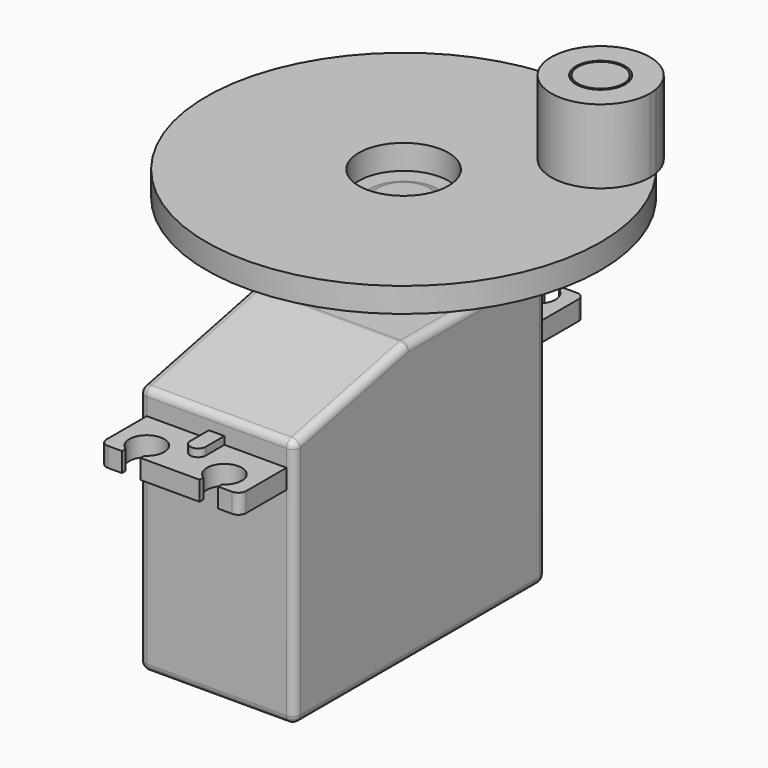
from build123d import *

# Parameters (mm, degrees)
F1_DEPTH  = 10
F0_W      = 7.5
F0_H      = 2.5
F2_DEPTH  = 9
F4_DEPTH  = 25
F5_W      = 2
F5_H      = 46.5
F6_DEPTH  = 1
F9_R      = 0.8128
F10_DEPTH = 2
F11_R     = 26.294756744
F12_DEPTH = 2
F13_R     = 0.99999
F14_R     = 25.4
F14_R_2   = 5.77
F15_DEPTH = 3.175
F16_R     = 2.921
F17_DEPTH = 9.525
F18_R     = 3.175
F19_DEPTH = 9.525


# Not quite as in the source:
# - a fillet or chamfer is up to 0.001 mm smaller than in the source, because OpenCascade refuses the exact size


with BuildPart() as f1:
    # F0 (on Right) → F1 (new body, symmetric)
    with BuildSketch(Plane.YZ):
        Polygon((-20.25, 26.6), (-20.25, 0), (20.25, 0), (20.25, 26.6), (20.25, 29.1), (20.25, 36.1), (-1.95, 36.1), (-20.25, 32.1), (-20.25, 29.1), align=None)
    extrude(amount=F1_DEPTH, both=True)

    # F0 (on Right) → F2 (join, symmetric)
    with BuildSketch(Plane.YZ):
        with Locations((-24, 27.85)):
            Rectangle(F0_W, F0_H)
        with Locations((24, 27.85)):
            Rectangle(F0_W, F0_H)
    extrude(amount=F2_DEPTH, both=True)

    # F3 (on face) → F4 (cut)
    with BuildSketch(Plane.XY.offset(29.1)):
        with BuildLine():
            ThreePointArc((-3.8, -27.1532866311), (-3.0299111695, -26.336853256), (-2.75, -25.25))
            ThreePointArc((-2.75, -25.25), (-6.086853256, -23.2799111695), (-6.2, -27.1532866311))
            ThreePointArc((-6.2, -27.1532866311), (-5, -27.5), (-3.8, -27.1532866311))
        make_face()
        with BuildLine():
            ThreePointArc((-3.8, -27.1532866311), (-5, -27.5), (-6.2, -27.1532866311))
            Line((-6.2, -27.1532866311), (-6.2, -27.75))
            Line((-6.2, -27.75), (-3.8, -27.75))
            Line((-3.8, -27.75), (-3.8, -27.1532866311))
        make_face()
        with BuildLine():
            Line((-3.8, 27.75), (-6.2, 27.75))
            Line((-6.2, 27.75), (-6.2, 27.1532866311))
            ThreePointArc((-6.2, 27.1532866311), (-5, 27.5), (-3.8, 27.1532866311))
            Line((-3.8, 27.1532866311), (-3.8, 27.75))
        make_face()
        with BuildLine():
            ThreePointArc((-3.8, 27.1532866311), (-5, 27.5), (-6.2, 27.1532866311))
            ThreePointArc((-6.2, 27.1532866311), (-6.086853256, 23.2799111695), (-2.75, 25.25))
            ThreePointArc((-2.75, 25.25), (-3.0299111695, 26.336853256), (-3.8, 27.1532866311))
        make_face()
        with BuildLine():
            Line((3.8, -27.1532866311), (3.8, -27.75))
            Line((3.8, -27.75), (6.2, -27.75))
            Line((6.2, -27.75), (6.2, -27.1532866311))
            ThreePointArc((6.2, -27.1532866311), (5, -27.5), (3.8, -27.1532866311))
        make_face()
        with BuildLine():
            ThreePointArc((7.25, -25.25), (3.913146744, -23.2799111695), (3.8, -27.1532866311))
            ThreePointArc((3.8, -27.1532866311), (5, -27.5), (6.2, -27.1532866311))
            ThreePointArc((6.2, -27.1532866311), (6.9700888305, -26.336853256), (7.25, -25.25))
        make_face()
        with BuildLine():
            Line((6.2, 27.75), (3.8, 27.75))
            Line((3.8, 27.75), (3.8, 27.1532866311))
            ThreePointArc((3.8, 27.1532866311), (5, 27.5), (6.2, 27.1532866311))
            Line((6.2, 27.1532866311), (6.2, 27.75))
        make_face()
        with BuildLine():
            ThreePointArc((6.2, 27.1532866311), (5, 27.5), (3.8, 27.1532866311))
            ThreePointArc((3.8, 27.1532866311), (3.913146744, 23.2799111695), (7.25, 25.25))
            ThreePointArc((7.25, 25.25), (6.9700888305, 26.336853256), (6.2, 27.1532866311))
        make_face()
    extrude(amount=-F4_DEPTH, mode=Mode.SUBTRACT)

    # F5 (on face) → F6 (join)
    with BuildSketch(Plane.XY.offset(29.1)):
        Rectangle(F5_W, F5_H)
        with BuildLine():
            Line((-1, 23.25), (1, 23.25))
            ThreePointArc((1, 23.25), (0, 24.25), (-1, 23.25))
        make_face()
        with BuildLine():
            ThreePointArc((-1, -23.25), (0, -24.25), (1, -23.25))
            Line((1, -23.25), (-1, -23.25))
        make_face()
    extrude(amount=F6_DEPTH)

    # F7 (on Right) → F8 (revolve)
    with BuildSketch(Plane.YZ):
        Polygon((9.85, 36.1), (16.85, 36.1), (13.85, 37.6), (13.85, 42.1), (29.85, 42.1), (29.85, 44.1), (14.35, 44.1), (13.1, 44.6), (9.85, 44.6), align=None)
    revolve(axis=Axis((0, 9.85, 38.956922479), (0, 0, -1)))

    # F9 (on face) → F10 (cut, through all)
    with BuildSketch(Plane.XY.offset(44.1)):
        with Locations((0, 17.3)):
            Circle(F9_R)
        with Locations((0, 20.3)):
            Circle(F9_R)
        with Locations((0, 23.3)):
            Circle(F9_R)
        with Locations((0, 26.3)):
            Circle(F9_R)
        with Locations((-16.45, 9.85)):
            Circle(F9_R)
        with Locations((-13.45, 9.85)):
            Circle(F9_R)
        with Locations((-10.45, 9.85)):
            Circle(F9_R)
        with Locations((-7.45, 9.85)):
            Circle(F9_R)
        with Locations((0, -6.6)):
            Circle(F9_R)
        with Locations((0, -3.6)):
            Circle(F9_R)
        with Locations((0, -0.6)):
            Circle(F9_R)
        with Locations((0, 2.4)):
            Circle(F9_R)
        with Locations((16.45, 9.85)):
            Circle(F9_R)
        with Locations((13.45, 9.85)):
            Circle(F9_R)
        with Locations((10.45, 9.85)):
            Circle(F9_R)
        with Locations((7.45, 9.85)):
            Circle(F9_R)
    extrude(amount=-F10_DEPTH, mode=Mode.SUBTRACT)

    # F11 (on face) → F12 (cut, through all)
    with BuildSketch(Plane.XY.offset(44.1)):
        with Locations((0, 9.85)):
            Circle(F11_R)
        with BuildLine():
            ThreePointArc((-4.8436814511, 14.6936814511), (-4.0616110554, 15.7958081166), (-3.6873277698, 17.0943570425))
            Line((-3.6873277698, 17.0943570425), (-2.5, 27.6162423281))
            ThreePointArc((-2.5, 27.6162423281), (-1.6762811024, 29.2102108544), (0, 29.85))
            ThreePointArc((0, 29.85), (1.6762811024, 29.2102108544), (2.5, 27.6162423281))
            Line((2.5, 27.6162423281), (3.6873277698, 17.0943570425))
            ThreePointArc((3.6873277698, 17.0943570425), (4.0616110554, 15.7958081166), (4.8436814511, 14.6936814511))
            ThreePointArc((4.8436814511, 14.6936814511), (5.9458081166, 13.9116110554), (7.2443570425, 13.5373277698))
            Line((7.2443570425, 13.5373277698), (17.7662423281, 12.35))
            ThreePointArc((17.7662423281, 12.35), (19.3602108544, 11.5262811024), (20, 9.85))
            ThreePointArc((20, 9.85), (19.3602108544, 8.1737188976), (17.7662423281, 7.35))
            Line((17.7662423281, 7.35), (7.2443570425, 6.1626722302))
            ThreePointArc((7.2443570425, 6.1626722302), (5.9458081166, 5.7883889446), (4.8436814511, 5.0063185489))
            ThreePointArc((4.8436814511, 5.0063185489), (4.0616110554, 3.9041918834), (3.6873277698, 2.6056429575))
            Line((3.6873277698, 2.6056429575), (2.5, -7.9162423281))
            ThreePointArc((2.5, -7.9162423281), (1.6762811024, -9.5102108544), (0, -10.15))
            ThreePointArc((0, -10.15), (-1.6762811024, -9.5102108544), (-2.5, -7.9162423281))
            Line((-2.5, -7.9162423281), (-3.6873277698, 2.6056429575))
            ThreePointArc((-3.6873277698, 2.6056429575), (-4.0616110554, 3.9041918834), (-4.8436814511, 5.0063185489))
            ThreePointArc((-4.8436814511, 5.0063185489), (-5.9458081166, 5.7883889446), (-7.2443570425, 6.1626722302))
            Line((-7.2443570425, 6.1626722302), (-17.7662423281, 7.35))
            ThreePointArc((-17.7662423281, 7.35), (-19.3602108544, 8.1737188976), (-20, 9.85))
            ThreePointArc((-20, 9.85), (-19.3602108544, 11.5262811024), (-17.7662423281, 12.35))
            Line((-17.7662423281, 12.35), (-7.2443570425, 13.5373277698))
            ThreePointArc((-7.2443570425, 13.5373277698), (-5.9458081166, 13.9116110554), (-4.8436814511, 14.6936814511))
        make_face(mode=Mode.SUBTRACT)
    extrude(amount=-F12_DEPTH, mode=Mode.SUBTRACT)

    # F13 (radius 1 in the source; OpenCascade refuses exactly that, so slightly less here)
    f13_edges = [f1.edges().sort_by_distance(p)[0] for p in [
        (10, -20.25, 16.05),
        (10, 0, 0),
        (10, 20.25, 18.05),
        (10, 9.15, 36.1),
        (10, -11.1, 34.1),
        (-10, 0, 0),
        (-10, 20.25, 18.05),
        (-10, 9.15, 36.1),
        (-10, -11.1, 34.1),
        (-10, -20.25, 16.05),
        (0, -20.25, 0),
        (0, 20.25, 0),
        (0, -1.95, 36.1),
        (0, -20.25, 32.1),
        (0, 20.25, 36.1),
        (0, 2.85, 36.1),
        (9, -27.75, 27.85),
        (-9, -27.75, 27.85),
        (9, 27.75, 27.85),
        (-9, 27.75, 27.85),
    ]]
    fillet(f13_edges, radius=F13_R)


with BuildPart() as f15:
    # F14 (on face) → F15 (new body)
    with BuildSketch(Plane.XY.offset(44.6)):
        with Locations((0, 9.85)):
            Circle(F14_R)
        with Locations((0, 9.85)):
            Circle(F14_R_2, mode=Mode.SUBTRACT)
    extrude(amount=F15_DEPTH)

    # F16 (on face) → F17 (join)
    with BuildSketch(Plane.XY.offset(47.775)):
        with Locations((14.0990021101, 23.9490021101)):
            Circle(F16_R)
    extrude(amount=F17_DEPTH)


with BuildPart() as f19:
    # F18 (on face) → F19 (new body)
    with BuildSketch(Plane.XY.offset(47.775)):
        with BuildLine():
            ThreePointArc((15.194945462, 30.2037129882), (9.2368143163, 19.8646870074), (20.4490021101, 23.9490021101))
            ThreePointArc((20.4490021101, 23.9490021101), (20.4251349761, 24.4990411649), (20.3537129882, 25.044945462))
            ThreePointArc((20.3537129882, 25.044945462), (17.9605122421, 27.8105122421), (15.194945462, 30.2037129882))
        make_face()
        with Locations((14.0990021101, 23.9490021101)):
            Circle(F18_R, mode=Mode.SUBTRACT)
        with BuildLine():
            ThreePointArc((15.194945462, 30.2037129882), (17.9605122421, 27.8105122421), (20.3537129882, 25.044945462))
            ThreePointArc((20.3537129882, 25.044945462), (18.5891301706, 28.4391301706), (15.194945462, 30.2037129882))
        make_face()
    extrude(amount=F19_DEPTH)


solid = Compound([f1.part, f15.part, f19.part])
